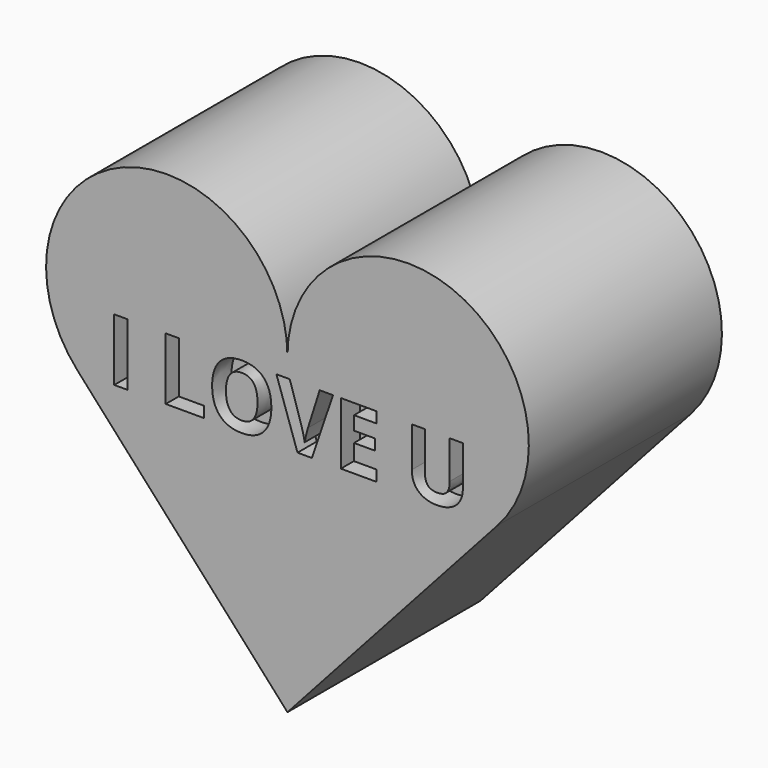
from build123d import *

# Parameters (mm, degrees)
F1_DEPTH     = 50
F2_TEXT_SIZE = 18.0403653174
F3_DEPTH     = 5


# Not quite as in the source:
# - Text() gives the source's letters only with a copy of the font that has no kerning and outlines rounded to 1/6400 em; it was checked with that copy


with BuildPart() as f1:
    # F0 (on Front) → F1 (new body)
    with BuildSketch(Plane.XZ):
        with BuildLine():
            ThreePointArc((43.5567010309, -16.7525773196), (33.9744769827, 23.3336401551), (0, 0))
            Line((0, 0), (0, -65))
            Line((0, -65), (43.5567010309, -16.7525773196))
        make_face()
        with BuildLine():
            Line((0, -65), (0, 0))
            ThreePointArc((0, 0), (-33.9744769827, 23.3336401551), (-43.5567010309, -16.7525773196))
            Line((-43.5567010309, -16.7525773196), (0, -65))
        make_face()
    extrude(amount=F1_DEPTH)

    # F2 (on face) → F3 (cut)
    with BuildSketch(Plane.XZ.offset(50)):
        with Locations((-37.5, -16.9890630285)):
            Text('I LOVE U', F2_TEXT_SIZE, font='Open Sans', font_style=FontStyle.BOLD, text_align=(TextAlign.LEFT, TextAlign.BOTTOM))
    extrude(amount=-F3_DEPTH, mode=Mode.SUBTRACT)


solid = f1.part
